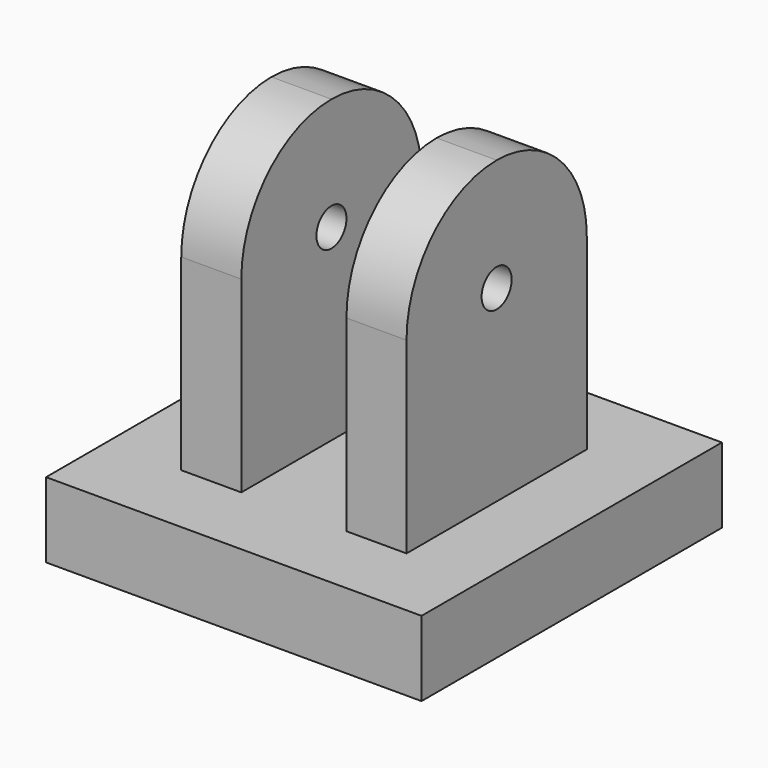
from build123d import *

# Parameters (mm, degrees)
F0_W     = 50
F0_H     = 50
F1_DEPTH = 10
F2_W     = 8
F2_H     = 30
F3_DEPTH = 50
F4_R     = 14.99999
F6_D     = 5


# Not quite as in the source:
# - a fillet or chamfer is up to 0.001 mm smaller than in the source, because OpenCascade refuses the exact size


with BuildPart() as f1:
    # F0 (on Top) → F1 (new body)
    with BuildSketch(Plane.XY):
        with Locations((-3.5858808544, -2.0939260721)):
            Rectangle(F0_W, F0_H)
    extrude(amount=F1_DEPTH)

    # F2 (on Top) → F3 (join)
    with BuildSketch(Plane.XY):
        with Locations((-14.5858808544, -2.0939260721)):
            Rectangle(F2_W, F2_H)
        with Locations((7.4141191456, -2.0939260721)):
            Rectangle(F2_W, F2_H)
    extrude(amount=F3_DEPTH)

    # F4 (radius 15 in the source; OpenCascade refuses exactly that, so slightly less here)
    f4_edges = [f1.edges().sort_by_distance(p)[0] for p in [
        (-14.585881, -17.093926, 50),
        (-14.585881, 12.906074, 50),
        (7.414119, -17.093926, 50),
        (7.414119, 12.906074, 50),
    ]]
    fillet(f4_edges, radius=F4_R)

    # F6 (through all)
    with Locations(Plane.YZ.offset(11.4141191456)):
        with Locations((-2.0939260721, 35)):
            Hole(F6_D / 2)


solid = f1.part
